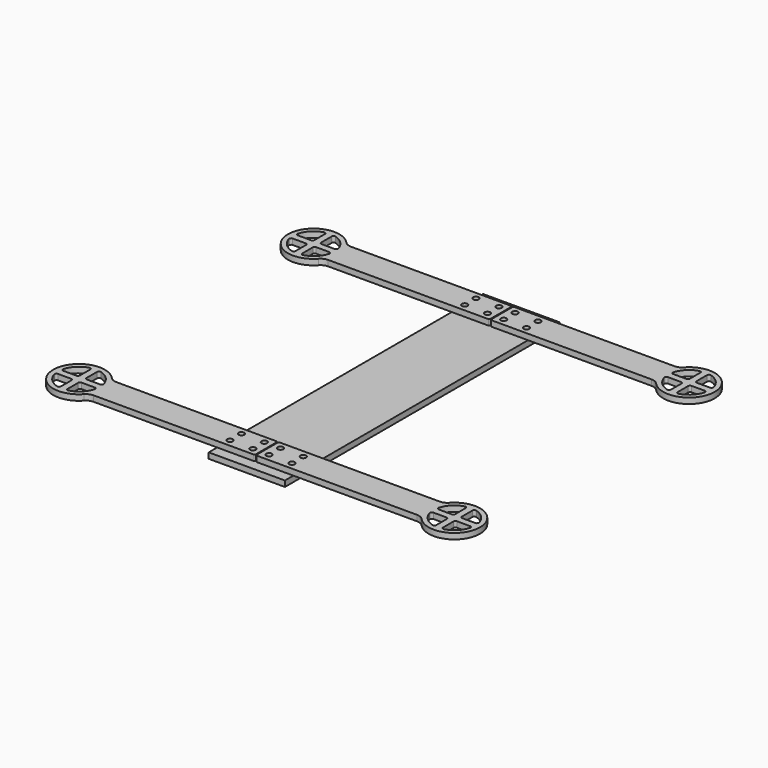
from build123d import *

# Parameters (mm, degrees)
F2_DEPTH         = 3
F3_R             = 1.5
F4_DEPTH         = 3
F4_COPIES2_COUNT = 2
F5_R             = 1.5
F6_DEPTH         = 3


# Not quite as in the source:
# - a pattern or mirror of a feature is missing from the dataset's text; its kind, count and spacing are read off the source's solid
# - a feature names something its author has since deleted; it is built from what else it names


with BuildPart() as f2:
    # F1 (on Top) → F2 (new body)
    with BuildSketch(Plane.XY):
        Polygon((0, 90), (-20, 90), (-20, -90), (0, -90), (20, -90), (20, 90), align=None)
    extrude(amount=F2_DEPTH)

    # F3 (on face) → F4 (join)
    with BuildSketch(Plane.XY.offset(3)):
        with BuildLine():
            ThreePointArc((-84.8631625039, 84.4576844157), (-86.8766306695, 84.8810103017), (-88.5491575571, 86.0793060373))
            ThreePointArc((-88.5491575571, 86.0793060373), (-112.0013442008, 76.9576844157), (-88.5491575571, 67.8360627941))
            ThreePointArc((-88.5491575571, 67.8360627941), (-86.8766306695, 69.0343585297), (-84.8631625039, 69.4576844157))
            Line((-84.8631625039, 69.4576844157), (-0.75, 69.4576844157))
            ThreePointArc((-0.75, 69.4576844157), (-0.3964466094, 69.6041310251), (-0.25, 69.9576844157))
            Line((-0.25, 69.9576844157), (-0.25, 83.9576844157))
            ThreePointArc((-0.25, 83.9576844157), (-0.3964466094, 84.3112378063), (-0.75, 84.4576844157))
            Line((-0.75, 84.4576844157), (-84.8631625039, 84.4576844157))
        make_face()
        with BuildLine():
            ThreePointArc((-109.0772306885, 73.9326844157), (-108.9142224335, 74.8097641446), (-108.1157864624, 75.2076844157))
            Line((-108.1157864624, 75.2076844157), (-101.2513442008, 75.2076844157))
            ThreePointArc((-101.2513442008, 75.2076844157), (-100.5442374197, 74.9147911969), (-100.2513442008, 74.2076844157))
            Line((-100.2513442008, 74.2076844157), (-100.2513442008, 67.3432421542))
            ThreePointArc((-100.2513442008, 67.3432421542), (-100.6492644719, 66.5448061831), (-101.5263442008, 66.381797928))
            ThreePointArc((-101.5263442008, 66.381797928), (-106.2795187939, 69.1795098227), (-109.0772306885, 73.9326844157))
        make_face(mode=Mode.SUBTRACT)
        with BuildLine():
            ThreePointArc((-87.9254577132, 73.9326844157), (-90.7231696078, 69.1795098227), (-95.4763442008, 66.381797928))
            ThreePointArc((-95.4763442008, 66.381797928), (-96.3534239298, 66.5448061831), (-96.7513442008, 67.3432421542))
            Line((-96.7513442008, 67.3432421542), (-96.7513442008, 74.2076844157))
            ThreePointArc((-96.7513442008, 74.2076844157), (-96.458450982, 74.9147911969), (-95.7513442008, 75.2076844157))
            Line((-95.7513442008, 75.2076844157), (-88.8869019393, 75.2076844157))
            ThreePointArc((-88.8869019393, 75.2076844157), (-88.0884659682, 74.8097641446), (-87.9254577132, 73.9326844157))
        make_face(mode=Mode.SUBTRACT)
        with Locations((-16.25, 73.2076844157)):
            Circle(F3_R, mode=Mode.SUBTRACT)
        with Locations((-4.25, 73.2076844157)):
            Circle(F3_R, mode=Mode.SUBTRACT)
        with BuildLine():
            ThreePointArc((-109.0772306885, 79.9826844157), (-106.2795187939, 84.7358590088), (-101.5263442008, 87.5335709034))
            ThreePointArc((-101.5263442008, 87.5335709034), (-100.6492644719, 87.3705626484), (-100.2513442008, 86.5721266772))
            Line((-100.2513442008, 86.5721266772), (-100.2513442008, 79.7076844157))
            ThreePointArc((-100.2513442008, 79.7076844157), (-100.5442374197, 79.0005776345), (-101.2513442008, 78.7076844157))
            Line((-101.2513442008, 78.7076844157), (-108.1157864624, 78.7076844157))
            ThreePointArc((-108.1157864624, 78.7076844157), (-108.9142224335, 79.1056046868), (-109.0772306885, 79.9826844157))
        make_face(mode=Mode.SUBTRACT)
        with BuildLine():
            Line((-96.7513442008, 79.7076844157), (-96.7513442008, 86.5721266772))
            ThreePointArc((-96.7513442008, 86.5721266772), (-96.3534239298, 87.3705626484), (-95.4763442008, 87.5335709034))
            ThreePointArc((-95.4763442008, 87.5335709034), (-90.7231696078, 84.7358590088), (-87.9254577132, 79.9826844157))
            ThreePointArc((-87.9254577132, 79.9826844157), (-88.0884659682, 79.1056046868), (-88.8869019393, 78.7076844157))
            Line((-88.8869019393, 78.7076844157), (-95.7513442008, 78.7076844157))
            ThreePointArc((-95.7513442008, 78.7076844157), (-96.458450982, 79.0005776345), (-96.7513442008, 79.7076844157))
        make_face(mode=Mode.SUBTRACT)
        with Locations((-16.25, 80.7076844157)):
            Circle(F3_R, mode=Mode.SUBTRACT)
        with Locations((-4.25, 80.7076844157)):
            Circle(F3_R, mode=Mode.SUBTRACT)
    f4 = extrude(amount=F4_DEPTH)

    # F4_copies: F4 across plane
    add(f4.mirror(Plane(origin=(0, 0, 0), x_dir=(0, 0, -1), z_dir=(0, -1, 0))))

    # F4_copies1: F4 across plane
    add(f4.mirror(Plane(origin=(0, 0, 0), x_dir=(0, 0, 1), z_dir=(1, 0, 0))))

    # F4_copies2: F4 ×2 about axis
    f4_copies2_axis = Axis((0, 0, 0), (0, 0, 1))
    for i in range(1, F4_COPIES2_COUNT):
        add(f4.rotate(f4_copies2_axis, i * 360 / F4_COPIES2_COUNT))

    # F5 (on face) → F6 (cut, through all)
    with BuildSketch(Plane.XY.offset(3)):
        with Locations((-16.25, 80.7076844157)):
            Circle(F5_R)
        with Locations((-4.25, 80.7076844157)):
            Circle(F5_R)
        with Locations((-4.25, 73.2076844157)):
            Circle(F5_R)
        with Locations((-16.25, 73.2076844157)):
            Circle(F5_R)
        with Locations((4.25, 80.7076844157)):
            Circle(F5_R)
        with Locations((16.25, 80.7076844157)):
            Circle(F5_R)
        with Locations((16.25, 73.2076844157)):
            Circle(F5_R)
        with Locations((4.25, 73.2076844157)):
            Circle(F5_R)
        with Locations((4.25, -73.2076844157)):
            Circle(F5_R)
        with Locations((16.25, -73.2076844157)):
            Circle(F5_R)
        with Locations((16.25, -80.7076844157)):
            Circle(F5_R)
        with Locations((4.25, -80.7076844157)):
            Circle(F5_R)
        with Locations((-4.25, -80.7076844157)):
            Circle(F5_R)
        with Locations((-4.25, -73.2076844157)):
            Circle(F5_R)
        with Locations((-16.25, -73.2076844157)):
            Circle(F5_R)
        with Locations((-16.25, -80.7076844157)):
            Circle(F5_R)
    extrude(amount=-F6_DEPTH, mode=Mode.SUBTRACT)


solid = f2.part
